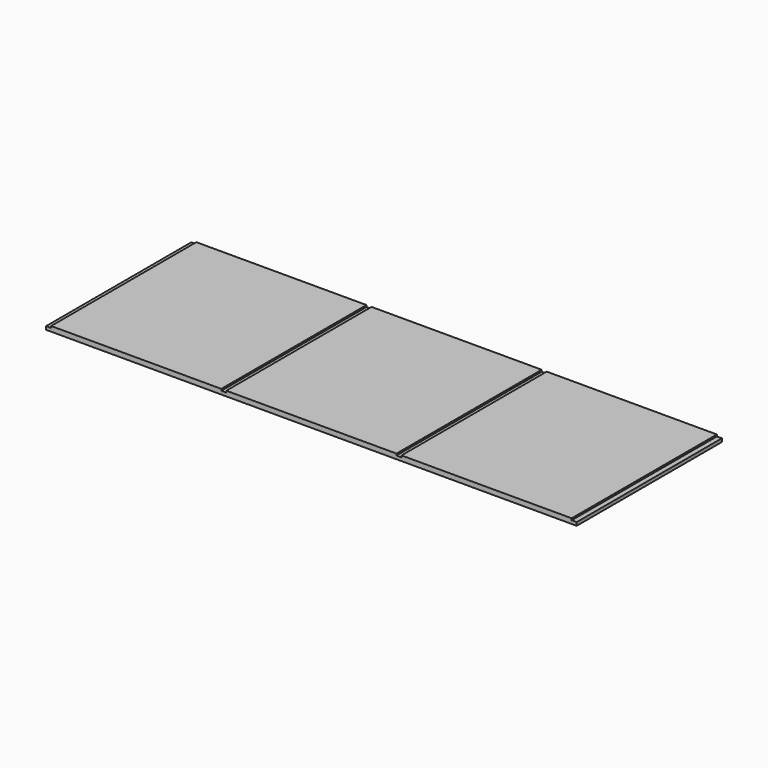
from build123d import *

# Parameters (mm, degrees)
F0_W     = 1930.4
F0_H     = 660.4
F1_DEPTH = 18.25625
F2_W     = 18.25625
F2_H     = 6.35
F3_DEPTH = 660.401
F4_W     = 18.25625
F4_H     = 6.35
F5_DEPTH = 660.401
F6_W     = 18.25625
F6_H     = 6.35
F7_DEPTH = 660.401
F8_W     = 18.25625
F8_H     = 6.35
F9_DEPTH = 660.401


# Not quite as in the source:
# - a length typed as a fraction of an inch, garbled in the dataset ("3 / 203.2 mm" for 3/8 in), is restored


with BuildPart() as f1:
    # F0 (on Top) → F1 (new body)
    with BuildSketch(Plane.XY):
        with Locations((302.4911884634, -5.2036456764)):
            Rectangle(F0_W, F0_H)
    extrude(amount=-F1_DEPTH)

    # F2 (on face) → F3 (cut, through all)
    with BuildSketch(Plane.XZ.offset(335.4036456764)):
        with Locations((-653.5806865366, -3.175)):
            Rectangle(F2_W, F2_H)
    extrude(amount=-F3_DEPTH, mode=Mode.SUBTRACT)

    # F4 (on face) → F5 (cut, through all)
    with BuildSketch(Plane.XZ.offset(335.4036456764)):
        with Locations((1258.5630634634, -3.175)):
            Rectangle(F4_W, F4_H)
    extrude(amount=-F5_DEPTH, mode=Mode.SUBTRACT)

    # F6 (on face) → F7 (cut, through all)
    with BuildSketch(Plane.XZ.offset(335.4036456764)):
        with Locations((621.1818134634, -3.175)):
            Rectangle(F6_W, F6_H)
    extrude(amount=-F7_DEPTH, mode=Mode.SUBTRACT)

    # F8 (on face) → F9 (cut, through all)
    with BuildSketch(Plane.XZ.offset(335.4036456764)):
        with Locations((-16.1994365366, -3.175)):
            Rectangle(F8_W, F8_H)
    extrude(amount=-F9_DEPTH, mode=Mode.SUBTRACT)


solid = f1.part
